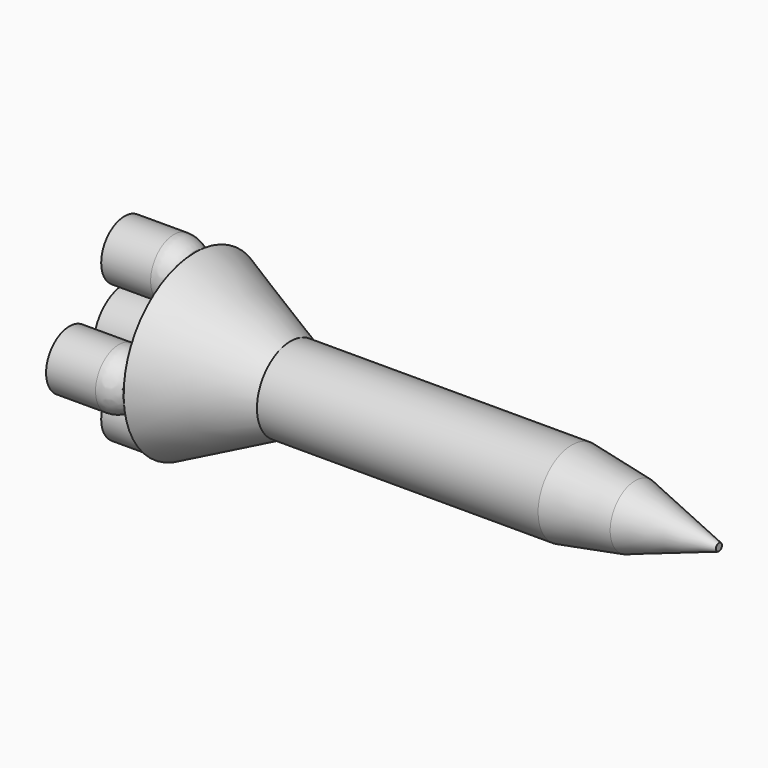
from build123d import *

# Parameters (mm, degrees)
F2_R       = 10.7168928343
F2_R_2     = 2.7397464127
F3_DEPTH   = 25
F4_SIZE    = 6.6
F5_SIZE    = 7.3
F6_DEPTH   = 25
F2_R_3     = 8.0928933426
F2_R_4     = 4.8185653545
F9_R       = 0.557922964
F9_2_R     = 0.557922964
F9_3_R     = 0.557922964
F9_4_R     = 0.557922964
F10_R      = 7.9
F10_2_R    = 7.9
F10_3_R    = 7.9
F10_4_R    = 7.9
F11_SIZE   = 3
F11_2_SIZE = 3
F11_3_SIZE = 3
F11_4_SIZE = 3


# Not quite as in the source:
# - a fillet or chamfer that OpenCascade refuses, or shapes differently, is made with other operations: its cross-section is extruded or revolved along the edge and cut away or added


with BuildPart() as f1:
    # F0 (on Front) → F1 (revolve)
    with BuildSketch(Plane.XZ):
        with BuildLine():
            ThreePointArc((56.7004742002, 0), (57.7038733342, 1.003399134), (58.7072724682, 0))
            Line((58.7072724682, 0), (65.7038733342, 0))
            Line((65.7038733342, 0), (65.7038733342, 1.0496124889))
            Line((65.7038733342, 1.0496124889), (42.4550920725, 8.6706466973))
            Line((42.4550920725, 8.6706466973), (24.8548462987, 11.6730295122))
            Line((24.8548462987, 11.6730295122), (-53.1934894355, 11.6730295122))
            Line((-53.1934894355, 11.6730295122), (-52.4483610687, 11.3070193437))
            Line((-52.4483610687, 11.3070193437), (-74.2961266658, 2.7397464127))
            Line((-74.2961266658, 2.7397464127), (-74.2961266658, 0))
            Line((-74.2961266658, 0), (56.7004742002, 0))
        make_face()
        with BuildLine():
            ThreePointArc((56.7004742002, 0), (57.7038733342, -1.003399134), (58.7072724682, 0))
            Line((58.7072724682, 0), (56.7004742002, 0))
        make_face()
        with BuildLine():
            Line((56.7004742002, 0), (58.7072724682, 0))
            ThreePointArc((58.7072724682, 0), (57.7038733342, 1.003399134), (56.7004742002, 0))
        make_face()
        Polygon((-79.760953784, 24.7230790555), (-74.2961266658, 2.7397464127), (-52.4483610687, 11.3070193437), (-53.4114667345, 11.6730295122), (-53.1934894355, 11.6730295122), align=None)
        Polygon((-53.4114667345, 11.6730295122), (-52.4483610687, 11.3070193437), (-53.1934894355, 11.6730295122), align=None)
    revolve(axis=Axis((-4.2961266658, 0, 0), (1, 0, 0)))


with BuildPart() as f3:
    # F2 (on face) → F3 (new body)
    with BuildSketch(Plane(origin=(-74.2961266658, 0, 0), x_dir=(0, -1, 0), z_dir=(-1, 0, 0))):
        Circle(F2_R)
        Circle(F2_R_2, mode=Mode.SUBTRACT)
    extrude(amount=F3_DEPTH)

    # F4
    f4_edges = [f3.edges().sort_by_distance(p)[0] for p in [
        (-99.296127, 2.739746, 0),
    ]]
    chamfer(f4_edges, length=F4_SIZE)

    # F5
    f5_edges = [f3.edges().sort_by_distance(p)[0] for p in [
        (-74.296127, 10.716893, 0),
    ]]
    chamfer(f5_edges, length=F5_SIZE)


with BuildPart() as f6:
    # F2 (on face) → F6 (new body)
    with BuildSketch(Plane(origin=(-74.2961266658, 0, 0), x_dir=(0, -1, 0), z_dir=(-1, 0, 0))):
        Circle(F2_R)
    extrude(amount=F6_DEPTH)


with BuildPart() as f6b:
    # F2 (on face) → F6, piece 2 (new body)
    with BuildSketch(Plane(origin=(-74.2961266658, 0, 0), x_dir=(0, -1, 0), z_dir=(-1, 0, 0))):
        with Locations((-19.1217530519, 0)):
            Circle(F2_R_3)
        with Locations((-19.1217530519, 0)):
            Circle(F2_R_4, mode=Mode.SUBTRACT)
    extrude(amount=F6_DEPTH)

    # F8#4: chamfer of 8 on 1 edges, made by hand

    # F8_4_s1 → F8_4_t2 (revolve, cut)
    with BuildSketch(Plane.XY):
        Polygon((-82.2961266658, 11.0288597092), (-74.2961266658, 19.0288597092), (-74.2961266658, 11.0288597092), align=None)
    revolve(axis=Axis((-74.2961266658, 19.1217530519, 0), (-1, 0, 0)), mode=Mode.SUBTRACT)

    # F9#4
    f9_4_edges = [f6b.edges().sort_by_distance(p)[0] for p in [
        (-79.021799, 23.940318, 0),
    ]]
    fillet(f9_4_edges, radius=F9_4_R)

    # F10#4
    f10_4_edges = [f6b.edges().sort_by_distance(p)[0] for p in [
        (-82.296127, 27.214646, 0),
    ]]
    fillet(f10_4_edges, radius=F10_4_R)

    # F11#2
    f11_2_edges = [f6b.edges().sort_by_distance(p)[0] for p in [
        (-99.296127, 23.940318, 0),
    ]]
    chamfer(f11_2_edges, length=F11_2_SIZE)


with BuildPart() as f6c:
    # F2 (on face) → F6, piece 3 (new body)
    with BuildSketch(Plane(origin=(-74.2961266658, 0, 0), x_dir=(0, -1, 0), z_dir=(-1, 0, 0))):
        with Locations((0, -19.1217530519)):
            Circle(F2_R_3)
        with Locations((0, -19.1217530519)):
            Circle(F2_R_4, mode=Mode.SUBTRACT)
    extrude(amount=F6_DEPTH)

    # F8#3: chamfer of 8 on 1 edges, made by hand

    # F8_3_s1 → F8_3_t2 (revolve, cut)
    with BuildSketch(Plane.XY.offset(-19.1217530519)):
        Polygon((-82.2961266658, -8.0928933426), (-74.2961266658, -0.0928933426), (-74.2961266658, -8.0928933426), align=None)
    revolve(axis=Axis((-74.2961266658, 0, -19.1217530519), (-1, 0, 0)), mode=Mode.SUBTRACT)

    # F9#3
    f9_3_edges = [f6c.edges().sort_by_distance(p)[0] for p in [
        (-79.021799, 4.818565, -19.121753),
    ]]
    fillet(f9_3_edges, radius=F9_3_R)

    # F10#3
    f10_3_edges = [f6c.edges().sort_by_distance(p)[0] for p in [
        (-81.13518, -6.931946, -19.121753),
        (-79.974233, 5.770974, -19.121753),
        (-82.296127, 8.092893, -19.121753),
    ]]
    fillet(f10_3_edges, radius=F10_3_R)

    # F11
    f11_edges = [f6c.edges().sort_by_distance(p)[0] for p in [
        (-99.296127, 4.818565, -19.121753),
    ]]
    chamfer(f11_edges, length=F11_SIZE)


with BuildPart() as f6d:
    # F2 (on face) → F6, piece 4 (new body)
    with BuildSketch(Plane(origin=(-74.2961266658, 0, 0), x_dir=(0, -1, 0), z_dir=(-1, 0, 0))):
        with Locations((19.1217530519, 0)):
            Circle(F2_R_3)
        with Locations((19.1217530519, 0)):
            Circle(F2_R_4, mode=Mode.SUBTRACT)
    extrude(amount=F6_DEPTH)

    # F8: chamfer of 8 on 1 edges, made by hand

    # F8_s1 → F8_t2 (revolve, cut)
    with BuildSketch(Plane.XY):
        Polygon((-82.2961266658, -27.2146463945), (-74.2961266658, -19.2146463945), (-74.2961266658, -27.2146463945), align=None)
    revolve(axis=Axis((-74.2961266658, -19.1217530519, 0), (-1, 0, 0)), mode=Mode.SUBTRACT)

    # F9
    f9_edges = [f6d.edges().sort_by_distance(p)[0] for p in [
        (-79.021799, -14.303188, 0),
    ]]
    fillet(f9_edges, radius=F9_R)

    # F10
    f10_edges = [f6d.edges().sort_by_distance(p)[0] for p in [
        (-81.13518, -26.053699, 0),
        (-79.974233, -13.350779, 0),
        (-82.296127, -11.02886, 0),
    ]]
    fillet(f10_edges, radius=F10_R)

    # F11#3
    f11_3_edges = [f6d.edges().sort_by_distance(p)[0] for p in [
        (-99.296127, -14.303188, 0),
    ]]
    chamfer(f11_3_edges, length=F11_3_SIZE)


with BuildPart() as f6e:
    # F2 (on face) → F6, piece 5 (new body)
    with BuildSketch(Plane(origin=(-74.2961266658, 0, 0), x_dir=(0, -1, 0), z_dir=(-1, 0, 0))):
        with Locations((0, 19.1217530519)):
            Circle(F2_R_3)
        with Locations((0, 19.1217530519)):
            Circle(F2_R_4, mode=Mode.SUBTRACT)
    extrude(amount=F6_DEPTH)

    # F8#2: chamfer of 8 on 1 edges, made by hand

    # F8_2_s1 → F8_2_t2 (revolve, cut)
    with BuildSketch(Plane.XY.offset(19.1217530519)):
        Polygon((-82.2961266658, -8.0928933426), (-74.2961266658, -0.0928933426), (-74.2961266658, -8.0928933426), align=None)
    revolve(axis=Axis((-74.2961266658, 0, 19.1217530519), (-1, 0, 0)), mode=Mode.SUBTRACT)

    # F9#2
    f9_2_edges = [f6e.edges().sort_by_distance(p)[0] for p in [
        (-79.021799, 4.818565, 19.121753),
    ]]
    fillet(f9_2_edges, radius=F9_2_R)

    # F10#2
    f10_2_edges = [f6e.edges().sort_by_distance(p)[0] for p in [
        (-82.296127, 8.092893, 19.121753),
    ]]
    fillet(f10_2_edges, radius=F10_2_R)

    # F11#4
    f11_4_edges = [f6e.edges().sort_by_distance(p)[0] for p in [
        (-99.296127, 4.818565, 19.121753),
    ]]
    chamfer(f11_4_edges, length=F11_4_SIZE)


solid = Compound([f1.part, f3.part, f6b.part, f6c.part, f6d.part, f6e.part])
